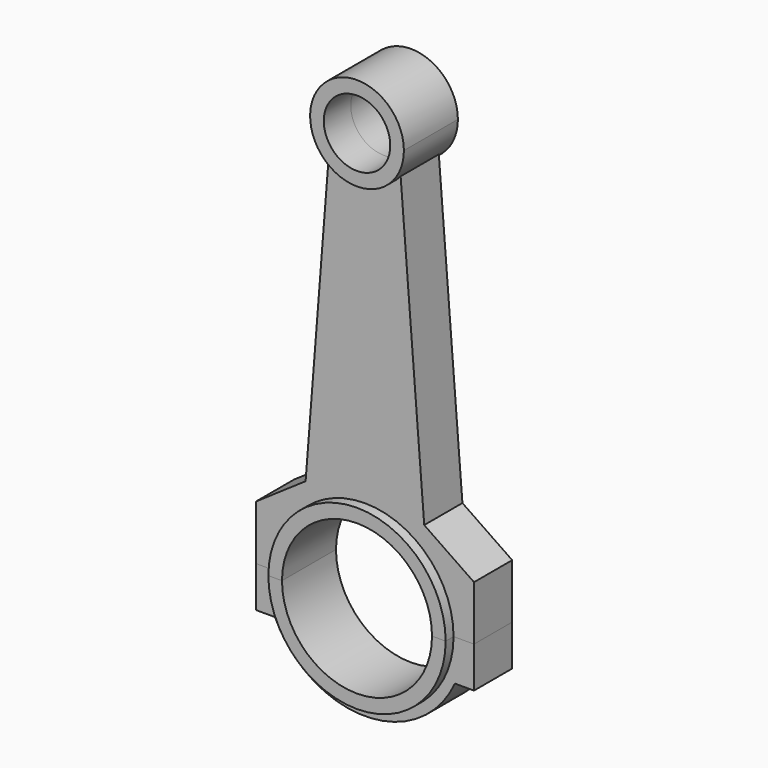
from build123d import *

# Parameters (mm, degrees)
F1_DEPTH = 12.573
F2_DEPTH = 8.89
F0_R     = 12.3825
F3_DEPTH = 12.573
F4_DEPTH = 12.573
F5_DEPTH = 8.89


with BuildPart() as f1:
    # F0 (on Front) → F1 (new body, symmetric)
    with BuildSketch(Plane.XZ):
        with BuildLine():
            ThreePointArc((-27.94, 0), (0, 27.94), (27.94, 0))
            Line((27.94, 0), (33.02, 0))
            ThreePointArc((33.02, 0), (0, 33.02), (-33.02, 0))
            Line((-33.02, 0), (-27.94, 0))
        make_face()
    extrude(amount=F1_DEPTH, both=True)

    # F0 (on Front) → F2 (join, symmetric)
    with BuildSketch(Plane.XZ):
        with BuildLine():
            ThreePointArc((-33.02, 0), (0, 33.02), (33.02, 0))
            Line((33.02, 0), (40.64, 0))
            Line((40.64, 0), (40.64, 20.32))
            Line((40.64, 20.32), (22.098, 33.02))
            Line((22.098, 33.02), (13.3114870458, 144.5266454276))
            ThreePointArc((13.3114870458, 144.5266454276), (0, 138.3665), (-13.3114870458, 144.5266454276))
            Line((-13.3114870458, 144.5266454276), (-22.098, 33.02))
            Line((-22.098, 33.02), (-40.64, 20.32))
            Line((-40.64, 20.32), (-40.64, 0))
            Line((-40.64, 0), (-33.02, 0))
        make_face()
    extrude(amount=F2_DEPTH, both=True)

    # F0 (on Front) → F3 (join, symmetric)
    with BuildSketch(Plane.XZ):
        with BuildLine():
            ThreePointArc((-13.3114870458, 144.5266454276), (0, 138.3665), (13.3114870458, 144.5266454276))
            ThreePointArc((13.3114870458, 144.5266454276), (16.3919301607, 149.8087398847), (17.4625, 155.829))
            ThreePointArc((17.4625, 155.829), (-6.0202601153, 172.2209301607), (-13.3114870458, 144.5266454276))
        make_face()
        with Locations((0, 155.829)):
            Circle(F0_R, mode=Mode.SUBTRACT)
    extrude(amount=F3_DEPTH, both=True)


with BuildPart() as f4:
    # F0 (on Front) → F4 (new body, symmetric)
    with BuildSketch(Plane.XZ):
        with BuildLine():
            Line((33.02, 0), (27.94, 0))
            ThreePointArc((27.94, 0), (0, -27.94), (-27.94, 0))
            Line((-27.94, 0), (-33.02, 0))
            ThreePointArc((-33.02, 0), (0, -33.02), (33.02, 0))
        make_face()
    extrude(amount=F4_DEPTH, both=True)

    # F0 (on Front) → F5 (join, symmetric)
    with BuildSketch(Plane.XZ):
        with BuildLine():
            Line((40.64, 0), (33.02, 0))
            ThreePointArc((33.02, 0), (0, -33.02), (-33.02, 0))
            Line((-33.02, 0), (-40.64, 0))
            Line((-40.64, 0), (-40.64, -15.24))
            Line((-40.64, -15.24), (-33.5289621074, -15.24))
            ThreePointArc((-33.5289621074, -15.24), (0, -36.83), (33.5289621074, -15.24))
            Line((33.5289621074, -15.24), (40.64, -15.24))
            Line((40.64, -15.24), (40.64, 0))
        make_face()
    extrude(amount=F5_DEPTH, both=True)


solid = Compound([f1.part, f4.part])
